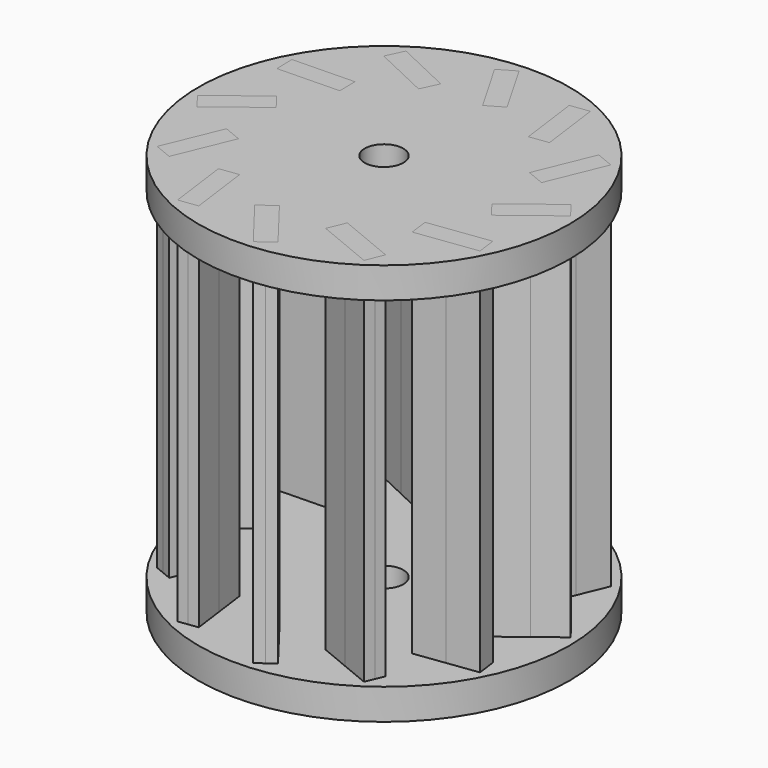
from build123d import *

# Parameters (mm, degrees)
F0_R        = 24
F0_R_2      = 2.5
F1_DEPTH    = 4
F2_DEPTH    = 52
F3_START    = 44
F1_FACE_R   = 24
F1_FACE_R_2 = 2.5
F3_DEPTH    = 4


# Not quite as in the source:
# - ends of sketch curves that miss each other by under 0.0002 mm in the source are joined


with BuildPart() as f1:
    # F0 (on Top) → F1 (new body)
    with BuildSketch(Plane.XY):
        Circle(F0_R)
        Polygon((-8.9827740816, -20.4386470385), (-10.2218230987, -20.6037455949), (-10.7501384793, -16.6387887403), (-11.2784538598, -12.6738318857), (-10.0394048428, -12.5087333293), (-8.8003558257, -12.3436347729), (-8.2720404452, -16.3085916275), (-7.7437250646, -20.273548482), align=None, mode=Mode.SUBTRACT)
        Polygon((-17.9994299012, -13.2083639741), (-19.154884362, -12.7314730129), (-17.6288332862, -9.0340187381), (-16.1027822104, -5.3365644633), (-14.9473277496, -5.8134554245), (-13.7918732887, -6.2903463857), (-15.3179243645, -9.9878006605), (-16.8439754403, -13.6852549352), align=None, mode=Mode.SUBTRACT)
        Polygon((-22.1901674017, -2.4646747911), (-22.9527062815, -1.4742029558), (-19.7513076007, 0.9904718354), (-16.613686535, 3.4060458753), (-15.8511476551, 2.4155740399), (-15.0886087753, 1.4251022046), (-18.226229841, -0.9904718354), (-21.4276285218, -3.4551466265), align=None, mode=Mode.SUBTRACT)
        Polygon((2.4405882298, -22.1931875166), (1.4490252381, -22.954309527), (-0.9915629917, -19.7851505161), (-3.4321512214, -16.6159915053), (-2.4405882298, -15.8548694949), (-1.4490252381, -15.0937474845), (0.9915629917, -18.2629064954), (3.4321512214, -21.4320655062), align=None, mode=Mode.SUBTRACT)
        Polygon((13.2082589659, -17.9995611772), (12.7313109402, -19.1549920841), (9.0339320379, -17.6287584019), (5.3365531356, -16.1025247196), (5.8135011613, -14.9470938127), (6.290449187, -13.7916629057), (9.9878280893, -15.3178965879), (13.6852069916, -16.8441302702), align=None, mode=Mode.SUBTRACT)
        Polygon((20.4379798112, -8.9871546743), (20.6014655966, -10.2264175189), (16.6358244939, -10.7495720322), (12.6701833913, -11.2727265454), (12.5066976059, -10.0334637008), (12.3432118205, -8.7942008562), (16.3088529232, -8.271046343), (20.2744940258, -7.7478918297), align=None, mode=Mode.SUBTRACT)
        Polygon((-20.3762131188, 9.3633951434), (-20.4049716149, 10.6130642792), (-16.4060303805, 10.7050914668), (-12.407089146, 10.7971186544), (-12.3783306499, 9.5474495186), (-12.3495721537, 8.2977803828), (-16.3485133882, 8.2057531952), (-20.3474546227, 8.1137260076), align=None, mode=Mode.SUBTRACT)
        Polygon((-13.1000797836, 18.1333488537), (-12.5662981354, 19.2636484388), (-8.9493394632, 17.5555471644), (-5.332380791, 15.84744589), (-5.8661624392, 14.7171463049), (-6.3999440875, 13.5868467198), (-10.0169027597, 15.2949479943), (-13.6338614319, 17.0030492687), align=None, mode=Mode.SUBTRACT)
        Circle(F0_R_2, mode=Mode.SUBTRACT)
        Polygon((22.1909529643, 2.4755624376), (22.9520749747, 1.4839994459), (19.737501164, -0.9915629917), (16.613756953, -3.3971770136), (15.8526349426, -2.4056140219), (15.0915129323, -1.4140510302), (18.2152571432, 0.9915629917), (21.4298309539, 3.4671254293), align=None, mode=Mode.SUBTRACT)
        Polygon((17.9982494725, 13.2093081016), (19.1539156294, 12.73293038), (17.6295069203, 9.0347986777), (16.1050982111, 5.3366669754), (14.9494320542, 5.813044697), (13.7937658972, 6.2894224186), (15.3181746063, 9.9875541209), (16.8425833155, 13.6856858232), align=None, mode=Mode.SUBTRACT)
        Polygon((8.9820708555, 20.4387540345), (10.2210853338, 20.6041115945), (10.7502295258, 16.6392652641), (11.2793737179, 12.6744189336), (10.0403592396, 12.5090613736), (8.8013447613, 12.3437038136), (8.2722005693, 16.3085501441), (7.7430563772, 20.2733964745), align=None, mode=Mode.SUBTRACT)
        Polygon((-2, 22.3566939084), (-0.9174682099, 22.9816938471), (1.0825317901, 19.517592232), (3.0825317901, 16.0534906169), (2, 15.4284906782), (0.9174682099, 14.8034907395), (-3.0825317901, 14.8034907395), (-3.0825317901, 21.7316939697), align=None, mode=Mode.SUBTRACT)
        Polygon((-1.0825317901, 18.2675923546), (-3.0825317901, 21.7316939697), (-3.0825317901, 14.8034907395), (0.9174682099, 14.8034907395), align=None)
    extrude(amount=F1_DEPTH)

    # F0 (on Top) → F2 (join)
    with BuildSketch(Plane.XY):
        Polygon((11.2793737179, 12.6744189336), (10.7502295258, 16.6392652641), (9.5112150476, 16.4739077041), (10.0403592396, 12.5090613736), align=None)
        Polygon((10.0403592396, 12.5090613736), (9.5112150476, 16.4739077041), (8.2722005693, 16.3085501441), (8.8013447613, 12.3437038136), align=None)
        Polygon((10.7502295258, 16.6392652641), (10.2210853338, 20.6041115945), (8.9820708555, 20.4387540345), (9.5112150476, 16.4739077041), align=None)
        Polygon((9.5112150476, 16.4739077041), (8.9820708555, 20.4387540345), (7.7430563772, 20.2733964745), (8.2722005693, 16.3085501441), align=None)
        Polygon((3.0825317901, 16.0534906169), (1.0825317901, 19.517592232), (0, 18.8925922933), (2, 15.4284906782), align=None)
        Polygon((2, 15.4284906782), (0, 18.8925922933), (-1.0825317901, 18.2675923546), (0.9174682099, 14.8034907395), align=None)
        Polygon((1.0825317901, 19.517592232), (-0.9174682099, 22.9816938471), (-2, 22.3566939084), (0, 18.8925922933), align=None)
        Polygon((0, 18.8925922933), (-2, 22.3566939084), (-3.0825317901, 21.7316939697), (-1.0825317901, 18.2675923546), align=None)
        Polygon((-8.9493394632, 17.5555471644), (-12.5662981354, 19.2636484388), (-13.1000797836, 18.1333488537), (-9.4831211114, 16.4252475793), align=None)
        Polygon((-9.4831211114, 16.4252475793), (-13.1000797836, 18.1333488537), (-13.6338614319, 17.0030492687), (-10.0169027597, 15.2949479943), align=None)
        Polygon((-5.332380791, 15.84744589), (-8.9493394632, 17.5555471644), (-9.4831211114, 16.4252475793), (-5.8661624392, 14.7171463049), align=None)
        Polygon((-5.8661624392, 14.7171463049), (-9.4831211114, 16.4252475793), (-10.0169027597, 15.2949479943), (-6.3999440875, 13.5868467198), align=None)
        Polygon((-12.407089146, 10.7971186544), (-16.4060303805, 10.7050914668), (-16.3772718843, 9.455422331), (-12.3783306499, 9.5474495186), align=None)
        Polygon((-16.4060303805, 10.7050914668), (-20.4049716149, 10.6130642792), (-20.3762131188, 9.3633951434), (-16.3772718843, 9.455422331), align=None)
        Polygon((-16.3772718843, 9.455422331), (-20.3762131188, 9.3633951434), (-20.3474546227, 8.1137260076), (-16.3485133882, 8.2057531952), align=None)
        Polygon((-12.3783306499, 9.5474495186), (-16.3772718843, 9.455422331), (-16.3485133882, 8.2057531952), (-12.3495721537, 8.2977803828), align=None)
        Polygon((-16.613686535, 3.4060458753), (-19.7513076007, 0.9904718354), (-18.9887687209, 0), (-15.8511476551, 2.4155740399), align=None)
        Polygon((-19.7513076007, 0.9904718354), (-22.9527062815, -1.4742029558), (-22.1901674017, -2.4646747911), (-18.9887687209, 0), align=None)
        Polygon((-18.9887687209, 0), (-22.1901674017, -2.4646747911), (-21.4276285218, -3.4551466265), (-18.226229841, -0.9904718354), align=None)
        Polygon((-15.8511476551, 2.4155740399), (-18.9887687209, 0), (-18.2262279469, -0.9904742957), (-15.0886087753, 1.4251022046), align=None)
        Polygon((-16.1027822104, -5.3365644633), (-17.6288332862, -9.0340187381), (-16.4733788254, -9.5109096993), (-14.9473277496, -5.8134554245), align=None)
        Polygon((-14.9473277496, -5.8134554245), (-16.4733788254, -9.5109096993), (-15.3179243645, -9.9878006605), (-13.7918732887, -6.2903463857), align=None)
        Polygon((-16.4733788254, -9.5109096993), (-17.9994299012, -13.2083639741), (-16.8439754403, -13.6852549352), (-15.3179243645, -9.9878006605), align=None)
        Polygon((-17.6288332862, -9.0340187381), (-19.154884362, -12.7314730129), (-17.9994299012, -13.2083639741), (-16.4733788254, -9.5109096993), align=None)
        Polygon((-10.7501384793, -16.6387887403), (-10.2218230987, -20.6037455949), (-8.9827740816, -20.4386470385), (-9.5110894622, -16.4736901839), align=None)
        Polygon((-9.5110894622, -16.4736901839), (-8.9827740816, -20.4386470385), (-7.7437250646, -20.273548482), (-8.2720404452, -16.3085916275), align=None)
        Polygon((-11.2784538598, -12.6738318857), (-10.7501384793, -16.6387887403), (-9.5110894622, -16.4736901839), (-10.0394048428, -12.5087333293), align=None)
        Polygon((-10.0394048428, -12.5087333293), (-9.5110894622, -16.4736901839), (-8.2720404452, -16.3085916275), (-8.8003558257, -12.3436347729), align=None)
        Polygon((-3.4321512214, -16.6159915053), (-0.9915629917, -19.7851505161), (0, -19.0240285057), (-2.4405882298, -15.8548694949), align=None)
        Polygon((-2.4405882298, -15.8548694949), (0, -19.0240285057), (0.9915629917, -18.2629064954), (-1.4490252381, -15.0937474845), align=None)
        Polygon((0, -19.0240285057), (2.4405882298, -22.1931875166), (3.4321512214, -21.4320655062), (0.9915629917, -18.2629064954), align=None)
        Polygon((-0.9915629917, -19.7851505161), (1.4490252381, -22.954309527), (2.4405882298, -22.1931875166), (0, -19.0240285057), align=None)
        Polygon((9.0339320379, -17.6287584019), (12.7313109402, -19.1549920841), (13.2082589659, -17.9995611772), (9.5108800636, -16.4733274949), align=None)
        Polygon((5.3365531356, -16.1025247196), (9.0339320379, -17.6287584019), (9.5108800636, -16.4733274949), (5.8135011613, -14.9470938127), align=None)
        Polygon((5.8135011613, -14.9470938127), (9.5108800636, -16.4733274949), (9.9878280893, -15.3178965879), (6.290449187, -13.7916629057), align=None)
        Polygon((9.5108800636, -16.4733274949), (13.2082589659, -17.9995611772), (13.6852069916, -16.8441302702), (9.9878280893, -15.3178965879), align=None)
        Polygon((12.6701833913, -11.2727265454), (16.6358244939, -10.7495720322), (16.4723387086, -9.5103091876), (12.5066976059, -10.0334637008), align=None)
        Polygon((16.6358244939, -10.7495720322), (20.6014655966, -10.2264175189), (20.4379798112, -8.9871546743), (16.4723387086, -9.5103091876), align=None)
        Polygon((12.5066976059, -10.0334637008), (16.4723387086, -9.5103091876), (16.3088529232, -8.271046343), (12.3432118205, -8.7942008562), align=None)
        Polygon((16.4723387086, -9.5103091876), (20.4379798112, -8.9871546743), (20.2744940258, -7.7478918297), (16.3088529232, -8.271046343), align=None)
        Polygon((16.613756953, -3.3971770136), (19.737501164, -0.9915629917), (18.9763791536, 0), (15.8526349426, -2.4056140219), align=None)
        Polygon((19.737501164, -0.9915629917), (22.9520749747, 1.4839994459), (22.1909529643, 2.4755624376), (18.9763791536, 0), align=None)
        Polygon((18.9763791536, 0), (22.1909529643, 2.4755624376), (21.4298309539, 3.4671254293), (18.2152571432, 0.9915629917), align=None)
        Polygon((15.8526349426, -2.4056140219), (18.9763791536, 0), (18.2152571432, 0.9915629917), (15.0915129323, -1.4140510302), align=None)
        Polygon((16.1050982111, 5.3366669754), (17.6295069203, 9.0347986777), (16.4738407633, 9.5111763993), (14.9494320542, 5.813044697), align=None)
        Polygon((14.9494320542, 5.813044697), (16.4738407633, 9.5111763993), (15.3181746063, 9.9875541209), (13.7937658972, 6.2894224186), align=None)
        Polygon((16.4738407633, 9.5111763993), (17.9982494725, 13.2093081016), (16.8425833155, 13.6856858232), (15.3181746063, 9.9875541209), align=None)
        Polygon((17.6295069203, 9.0347986777), (19.1539156294, 12.73293038), (17.9982494725, 13.2093081016), (16.4738407633, 9.5111763993), align=None)
    extrude(amount=F2_DEPTH)


with BuildPart() as f3:
    # F1_face (on face) → F3 (new body)
    with BuildSketch(Plane(origin=(-0.0016074104, 0.0028842551, 4), x_dir=(1, 0, 0), z_dir=(0, 0, 1)).offset(F3_START)):
        with Locations((0.0016074104, -0.0028842551)):
            Circle(F1_FACE_R)
        Polygon((-7.7421176542, -20.2764327371), (-10.2202156883, -20.60662985), (-11.2768464494, -12.6767161408), (-8.7987484153, -12.346519028), align=None, mode=Mode.SUBTRACT)
        Polygon((-16.8423680298, -13.6881391903), (-19.1532769516, -12.734357268), (-16.1011748, -5.3394487184), (-13.7902658783, -6.2932306408), align=None, mode=Mode.SUBTRACT)
        Polygon((-18.2246224306, -0.9933560905), (-21.4260211114, -3.4580308816), (-22.9510988711, -1.4770872108), (-16.6120791246, 3.4031616202), (-15.0870013648, 1.4222179495), (-18.2246205365, -0.9933585508), align=None, mode=Mode.SUBTRACT)
        Polygon((3.4337586319, -21.4349497613), (1.4506326485, -22.9571937821), (-3.430543811, -16.6188757604), (-1.4474178276, -15.0966317396), align=None, mode=Mode.SUBTRACT)
        Polygon((13.6868144021, -16.8470145253), (12.7329183507, -19.1578763392), (5.3381605461, -16.1054089747), (6.2920565975, -13.7945471608), align=None, mode=Mode.SUBTRACT)
        with Locations((0.0016074104, -0.0028842551)):
            Circle(F1_FACE_R_2, mode=Mode.SUBTRACT)
        Polygon((20.2761014363, -7.7507760848), (20.6030730071, -10.229301774), (12.6717908017, -11.2756108005), (12.3448192309, -8.7970851113), align=None, mode=Mode.SUBTRACT)
        Polygon((-20.4033642045, 10.6101800241), (-12.4054817355, 10.7942343993), (-12.3479647433, 8.2948961277), (-20.3458472122, 8.1108417526), align=None, mode=Mode.SUBTRACT)
        Polygon((-13.6322540214, 17.0001650136), (-12.5646907249, 19.2607641837), (-5.3307733805, 15.8445616349), (-6.398336677, 13.5839624647), align=None, mode=Mode.SUBTRACT)
        Polygon((21.4314383644, 3.4642411742), (22.9536823851, 1.4811151908), (16.6153643635, -3.4000612687), (15.0931203427, -1.4169352853), align=None, mode=Mode.SUBTRACT)
        Polygon((16.8441907259, 13.6828015681), (19.1555230399, 12.7300461249), (16.1067056216, 5.3337827203), (13.7953733076, 6.2865381635), align=None, mode=Mode.SUBTRACT)
        Polygon((7.7446637877, 20.2705122194), (10.2226927442, 20.6012273394), (11.2809811283, 12.6715346785), (8.8029521718, 12.3408195585), align=None, mode=Mode.SUBTRACT)
        Polygon((-3.0809243797, 21.7288097146), (-0.9158607994, 22.978809592), (3.0841392006, 16.0506063618), (0.9190756203, 14.8006064844), align=None, mode=Mode.SUBTRACT)
    extrude(amount=F3_DEPTH)


solid = Compound([f1.part, f3.part])
